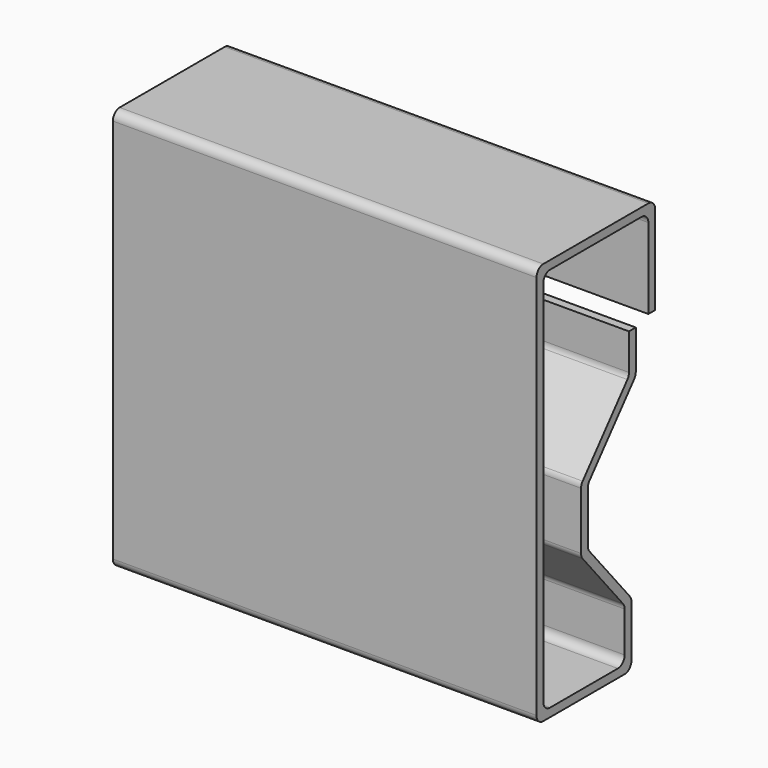
from build123d import *

# Parameters (mm, degrees)
F1_DEPTH = 100
F2_R     = 2


with BuildPart() as f1:
    # F0 (on Right) → F1 (new body)
    with BuildSketch(Plane.YZ):
        Polygon((33, -23), (35, -23), (35, 0), (0, 0), (0, -95), (28, -95), (28, -80), (15.1442478063, -64.6791111376), (15.1442478063, -51.1349920747), (29.2855752194, -34.2820143261), (29.2855752194, -24.2820143261), (27.2855752194, -24.2820143261), (27.2855752194, -33.5540738575), (13.1442478063, -50.4070516062), (13.1442478063, -65.4070516062), (26, -80.7279404685), (26, -93), (2, -93), (2, -2), (33, -2), align=None)
    extrude(amount=F1_DEPTH)

    # F2
    f2_edges = [f1.edges().sort_by_distance(p)[0] for p in [
        (50, 35, 0),
        (50, 0, 0),
        (50, 33, -2),
        (50, 2, -2),
        (50, 0, -95),
        (50, 28, -95),
        (50, 28, -80),
        (50, 29.285575, -34.282014),
        (50, 2, -93),
        (50, 26, -93),
        (50, 26, -80.72794),
        (50, 27.285575, -33.554074),
        (50, 15.144248, -64.679111),
        (50, 15.144248, -51.134992),
        (50, 13.144248, -50.407052),
        (50, 13.144248, -65.407052),
    ]]
    fillet(f2_edges, radius=F2_R)


solid = f1.part
